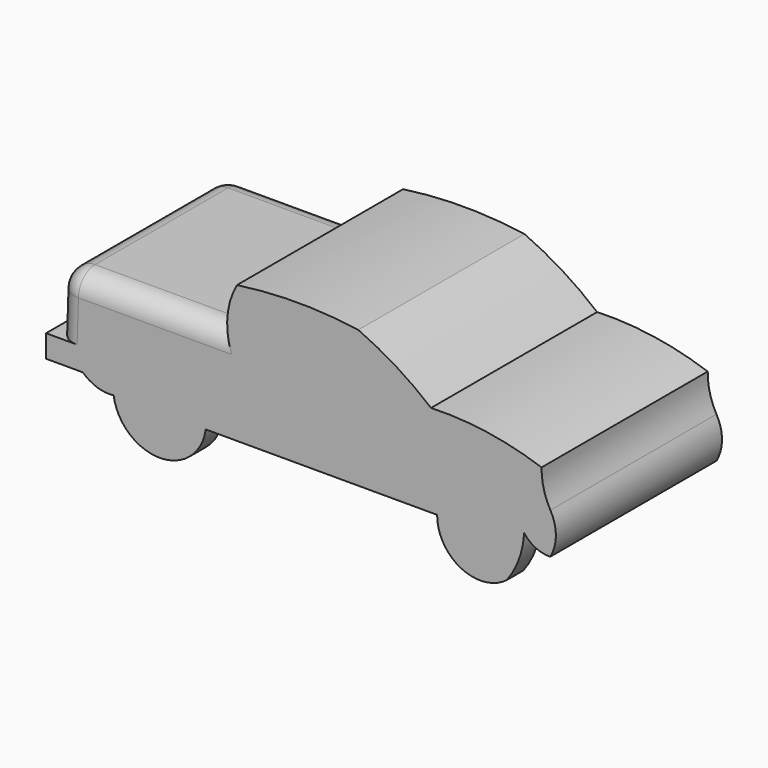
from build123d import *

# Parameters (mm, degrees)
F1_DEPTH     = 50.8
F2_W         = 100.3971769168
F2_H         = 40.64
F3_DEPTH     = 25.4
F5_R         = 5.08
F4_TEXT_SIZE = 5.9811271751
F6_DEPTH     = 0.254


# Not quite as in the source:
# - Text() gives the source's letters only with a copy of the font that has no kerning and outlines rounded to 1/6400 em; it was checked with that copy


with BuildPart() as f1:
    # F0 (on Front) → F1 (new body)
    with BuildSketch(Plane.XZ):
        with BuildLine():
            Line((-20.1590135694, 18.2808451355), (-61.4787340164, 18.2808451355))
            Line((-61.4787340164, 18.2808451355), (-61.9795769453, 3.0050706118))
            Line((-61.9795769453, 3.0050706118), (-64.4838064909, 3.0050706118))
            Line((-64.4838064909, 3.0050706118), (-64.4838064909, -2.5042253546))
            Line((-64.4838064909, -2.5042253546), (-55.4685927927, -2.5042253546))
            ThreePointArc((-55.4685927927, -2.5042253546), (-51.9917217828, -4.5947413495), (-47.9559153318, -5.0084507093))
            ThreePointArc((-47.9559153318, -5.0084507093), (-36.6869019344, -14.7997536644), (-25.417888537, -5.0084507093))
            Line((-25.417888537, -5.0084507093), (31.1776082963, -5.0084507093))
            ThreePointArc((31.1776082963, -5.0084507093), (37.0207636914, -14.5997317093), (48.1997533836, -13.5202292063))
            ThreePointArc((48.1997533836, -13.5202292063), (51.1910166517, -8.0799647059), (52.463516593, -2.0033803303))
            ThreePointArc((52.463516593, -2.0033803303), (55.2928693041, -4.2999364426), (58.8674202234, -5.0084507093))
            ThreePointArc((58.8674202234, -5.0084507093), (60.2117373378, 0), (58.8674202234, 5.0084507093))
            ThreePointArc((58.8674202234, 5.0084507093), (57.2294551617, 9.1232803706), (56.720700115, 13.5228168219))
            ThreePointArc((56.720700115, 13.5228168219), (43.3826008867, 16.7730344114), (29.6750683337, 17.5295770168))
            ThreePointArc((29.6750683337, 17.5295770168), (21.1746000008, 23.6674353013), (11.8950679898, 28.5481680185))
            ThreePointArc((11.8950679898, 28.5481680185), (-2.9521239572, 29.6125163479), (-17.7993159042, 28.5481680185))
            ThreePointArc((-17.7993159042, 28.5481680185), (-19.728005488, 23.5866096453), (-20.1590135694, 18.2808451355))
        make_face()
    extrude(amount=F1_DEPTH)

    # F2 (on face) → F3 (cut)
    with BuildSketch(Plane(origin=(0, 0, -5.0084507093), x_dir=(1, 0, 0), z_dir=(0, 0, -1))):
        with Locations((2.791043371, 25.4)):
            Rectangle(F2_W, F2_H)
    extrude(amount=F3_DEPTH, mode=Mode.SUBTRACT)

    # F5
    f5_edges = [f1.edges().sort_by_distance(p)[0] for p in [
        (-40.818874, -50.8, 18.280845),
        (-61.729155, -50.8, 10.642958),
        (-61.478734, -25.4, 18.280845),
        (-61.729155, 0, 10.642958),
        (-40.818874, 0, 18.280845),
    ]]
    fillet(f5_edges, radius=F5_R)

    # F4 (on face) → F6 (cut)
    with BuildSketch(Plane(origin=(-62.0114429478, 0, 2.0331533869), x_dir=(0, -1, 0), z_dir=(-0.9994629476, 0, 0.0327691371))):
        with Locations((3.81, 2.1603780345)):
            Text('Mason Hrdlicka', F4_TEXT_SIZE, font='Open Sans', text_align=(TextAlign.LEFT, TextAlign.BOTTOM))
    extrude(amount=-F6_DEPTH, mode=Mode.SUBTRACT)


solid = f1.part
